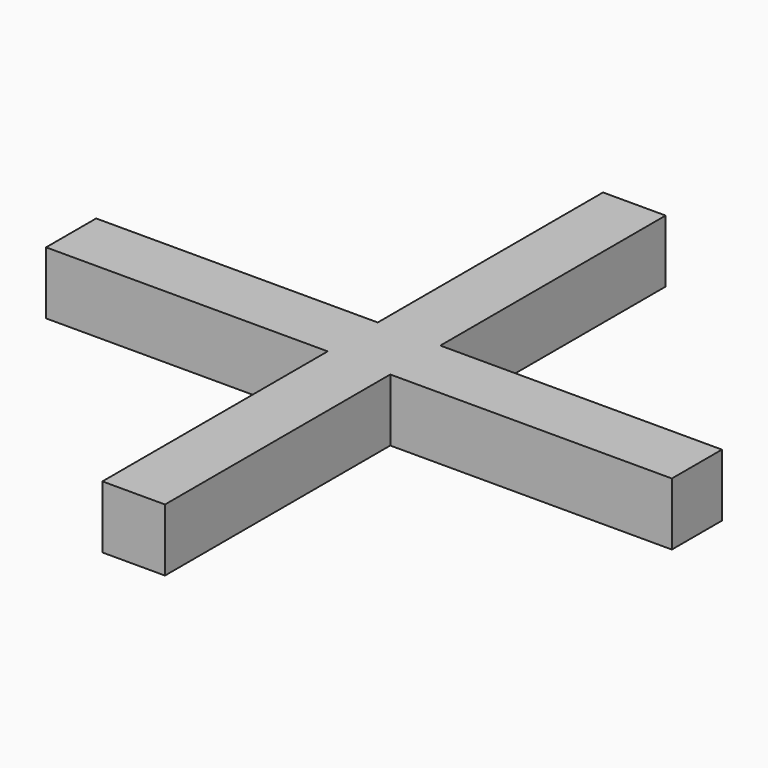
from build123d import *

# Parameters (mm, degrees)
F0_W     = 45
F0_H     = 10
F0_W_2   = 10
F0_H_2   = 45
F1_DEPTH = 10


# Not quite as in the source:
# - a feature of the source that left no trace in its solid (it failed there, or was rolled back) is left out


with BuildPart() as f1:
    # F0 (on Top) → F1 (new body)
    with BuildSketch(Plane.XY):
        with Locations((-27.5, 0)):
            Rectangle(F0_W, F0_H)
        with Locations((0, 27.5)):
            Rectangle(F0_W_2, F0_H_2)
        Rectangle(F0_W_2, F0_H)
        with Locations((27.5, 0)):
            Rectangle(F0_W, F0_H)
        with Locations((0, -27.5)):
            Rectangle(F0_W_2, F0_H_2)
    extrude(amount=F1_DEPTH)


solid = f1.part
